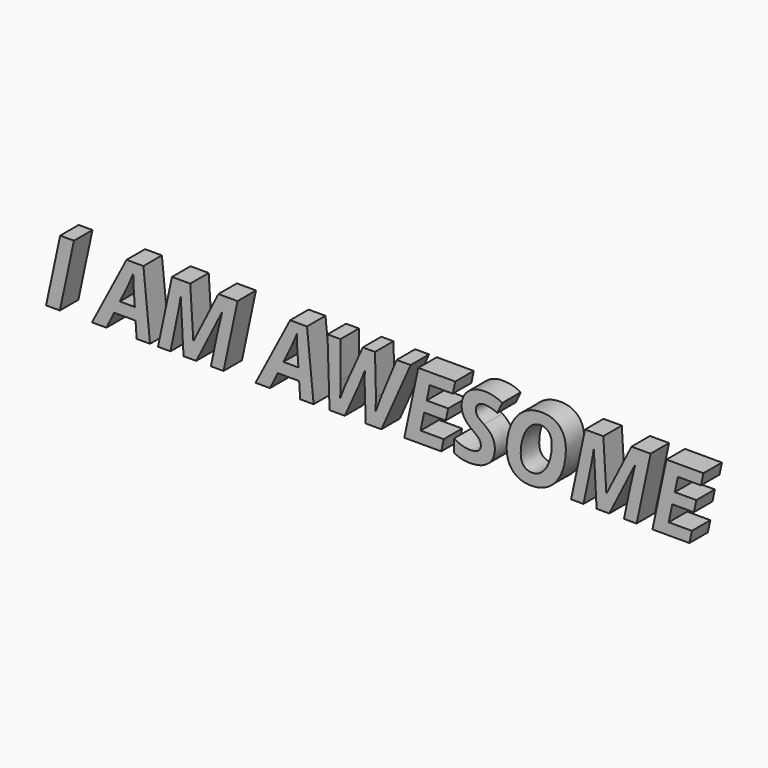
from build123d import *

# Parameters (mm, degrees)
F0_TEXT_SIZE = 1016.8711447881
F1_DEPTH     = 254


# Not quite as in the source:
# - Text() gives the source's letters only with a copy of the font that has no kerning and outlines rounded to 1/6400 em; it was checked with that copy


with BuildPart() as f1:
    # F0 (on Front) → F1 (new body)
    with BuildSketch(Plane.XZ):
        with Locations((-71.1113885045, -645.5227136612)):
            Text('I AM AWESOME', F0_TEXT_SIZE, font='Open Sans', font_style=FontStyle.BOLDITALIC, text_align=(TextAlign.LEFT, TextAlign.BOTTOM))
    extrude(amount=F1_DEPTH)


solid = f1.part
